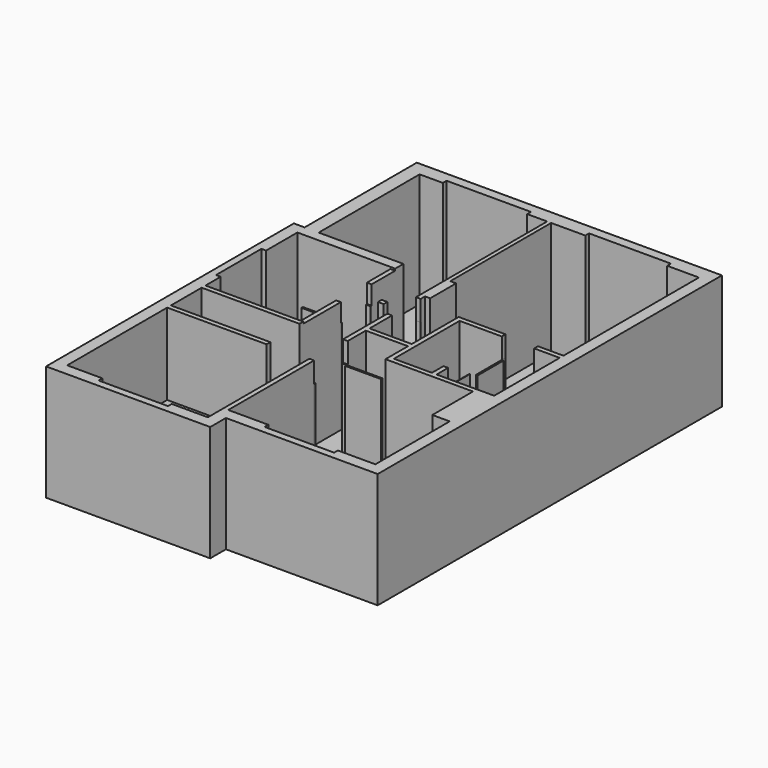
from build123d import *

# Parameters (mm, degrees)
F6_DEPTH  = 2440
F7_DEPTH  = 25
F8_DEPTH  = 2440
F2_W      = 100
F2_H      = 762
F9_DEPTH  = 3100
F3_W      = 690
F3_H      = 100
F10_DEPTH = 3100
F5_W      = 100
F5_H      = 1000
F5_H_2    = 627
F11_DEPTH = 2400
F12_W     = 10
F12_H     = 1000
F13_DEPTH = 2000
F14_W     = 600
F14_H     = 305
F15_DEPTH = 800
F18_DEPTH = 400
F19_W     = 600
F19_H     = 305
F20_DEPTH = 800
F22_DEPTH = 170
F23_W     = 30
F23_H     = 100
F24_DEPTH = 2000
F23_W_2   = 38
F23_H_2   = 762
F23_W_3   = 122
F25_W     = 100
F25_H     = 30
F26_DEPTH = 2000
F25_W_2   = 762
F25_H_2   = 38
F27_W     = 100
F27_H     = 30
F28_DEPTH = 2000
F27_W_2   = 762
F27_H_2   = 38
F29_W     = 760
F29_H     = 38
F30_DEPTH = 2000
F29_W_2   = 100
F29_H_2   = 30
F29_H_3   = 43.9612102509
F31_W     = 38
F31_H     = 690
F32_DEPTH = 2000
F31_W_2   = 30
F31_H_2   = 100
F33_W     = 1746.4833408594
F33_H     = 832.062959671
F34_DEPTH = 500
F35_W     = 906
F35_H     = 774.5329933167
F36_DEPTH = 706
F37_W     = 800
F37_H     = 1700
F38_DEPTH = 25
F40_DEPTH = 400


with BuildPart() as f6:
    # F0 (on Top) → F6 (new body)
    with BuildSketch(Plane.XY):
        Polygon((3250, -250), (3250, 168), (3704, 168), (5687, 168), (6486, 168), (6486, 2650), (6486, 3335), (6486, 9343), (775, 9343), (-20, 9343), (-20, 6353), (-250, 6353), (-250, -250), (499, -250), (2479, -250), align=None)
        Polygon((749, 0), (0, 0), (0, 2665), (6.1189043336, 2665), (2119, 2665), (2119, 2765), (0, 2765), (0, 3585), (2086, 3585), (2086, 3685), (1, 3685), (1, 4091), (-99, 4091), (-99, 5299), (1, 5299), (1, 6134), (2086, 6134), (2086, 6353), (280, 6353), (280, 9043), (775, 9043), (775, 9143), (2575, 9143), (2575, 9043), (3000, 9043), (3000, 3603), (3100, 3603), (3100, 5663), (3210, 5663), (3210, 6354), (3085, 6354), (3085, 9043), (3814, 9043), (3814, 9143), (5559, 9143), (5559, 9043), (6236, 9043), (6236, 3585), (5866, 3585), (5866, 2400), (6236, 2400), (6236, 418), (5437, 418), (5437, 318), (3954, 318), (3954, 418), (3100, 418), (3100, 2705), (3000, 2705), (3000, 0), (2229, 0), (2229, -100), (749, -100), align=None, mode=Mode.SUBTRACT)
    extrude(amount=F6_DEPTH)

    # F1 (on face) + F0 (on Top) → F7 (join)
    with BuildSketch(Plane.XY):
        Polygon((3100, 4183), (3100, 4083), (4000, 4083), (4000, 3483), (5866, 3483), (5866, 3583), (5010, 3583), (5010, 3890), (4910, 3890), (4910, 3583), (4100, 3583), (4100, 5333), (6236, 5333), (6236, 5433), (4000, 5433), (4000, 4183), align=None)
    with BuildSketch(Plane.XY):
        Polygon((3250, -250), (3250, 168), (3704, 168), (5687, 168), (6486, 168), (6486, 2650), (6486, 3335), (6486, 9343), (775, 9343), (-20, 9343), (-20, 6353), (-250, 6353), (-250, -250), (499, -250), (2479, -250), align=None)
        Polygon((749, 0), (0, 0), (0, 2665), (6.1189043336, 2665), (2119, 2665), (2119, 2765), (0, 2765), (0, 3585), (2086, 3585), (2086, 3685), (1, 3685), (1, 4091), (-99, 4091), (-99, 5299), (1, 5299), (1, 6134), (2086, 6134), (2086, 6353), (280, 6353), (280, 9043), (775, 9043), (775, 9143), (2575, 9143), (2575, 9043), (3000, 9043), (3000, 3603), (3100, 3603), (3100, 5663), (3210, 5663), (3210, 6354), (3085, 6354), (3085, 9043), (3814, 9043), (3814, 9143), (5559, 9143), (5559, 9043), (6236, 9043), (6236, 3585), (5866, 3585), (5866, 2400), (6236, 2400), (6236, 418), (5437, 418), (5437, 318), (3954, 318), (3954, 418), (3100, 418), (3100, 2705), (3000, 2705), (3000, 0), (2229, 0), (2229, -100), (749, -100), align=None, mode=Mode.SUBTRACT)
        Polygon((0, 2665), (0, 0), (749, 0), (749, -100), (2229, -100), (2229, 0), (3000, 0), (3000, 2705), (3100, 2705), (3100, 418), (3954, 418), (3954, 318), (5437, 318), (5437, 418), (6236, 418), (6236, 2400), (5866, 2400), (5866, 3585), (6236, 3585), (6236, 9043), (5559, 9043), (5559, 9143), (3814, 9143), (3814, 9043), (3085, 9043), (3085, 6354), (3210, 6354), (3210, 5663), (3100, 5663), (3100, 3603), (3000, 3603), (3000, 9043), (2575, 9043), (2575, 9143), (775, 9143), (775, 9043), (280, 9043), (280, 6353), (2086, 6353), (2086, 6134), (1, 6134), (1, 5299), (-99, 5299), (-99, 4091), (1, 4091), (1, 3685), (2086, 3685), (2086, 3585), (0, 3585), (0, 2765), (2119, 2765), (2119, 2665), (6.1189043336, 2665), align=None)
    extrude(amount=-F7_DEPTH)

    # F1 (on face) → F8 (join)
    with BuildSketch(Plane.XY):
        Polygon((3100, 4183), (3100, 4083), (4000, 4083), (4000, 3483), (5866, 3483), (5866, 3583), (5010, 3583), (5010, 3890), (4910, 3890), (4910, 3583), (4100, 3583), (4100, 5333), (6236, 5333), (6236, 5433), (4000, 5433), (4000, 4183), align=None)
    extrude(amount=F8_DEPTH)

    # F2 (on Top) → F9 (cut)
    with BuildSketch(Plane.XY):
        with Locations((3050, 5164)):
            Rectangle(F2_W, F2_H)
    extrude(amount=F9_DEPTH, mode=Mode.SUBTRACT)

    # F3 (on Top) → F10 (cut)
    with BuildSketch(Plane.XY):
        with Locations((5345, 5383)):
            Rectangle(F3_W, F3_H)
    extrude(amount=F10_DEPTH, mode=Mode.SUBTRACT)

    # F5 (on Top) → F11 (join)
    with BuildSketch(Plane.XY):
        with Locations((2036, 4185)):
            Rectangle(F5_W, F5_H)
        with Locations((2036, 5820.5)):
            Rectangle(F5_W, F5_H_2)
    extrude(amount=F11_DEPTH)

    # F12 (on Top) → F13 (join)
    with BuildSketch(Plane.XY):
        with Locations((4900, 4108)):
            Rectangle(F12_W, F12_H)
    extrude(amount=F13_DEPTH)

    # F14 (on Top) → F15 (join)
    with BuildSketch(Plane.XY):
        with Locations((5936, 3737.5)):
            Rectangle(F14_W, F14_H)
    extrude(amount=F15_DEPTH)

    # F17 (on Top) → F18 (join)
    with BuildSketch(Plane.XY):
        with BuildLine():
            ThreePointArc((5798.5, 4446), (5713.6471862576, 4410.8528137424), (5678.5, 4326))
            Line((5678.5, 4326), (5678.5, 3891))
            Line((5678.5, 3891), (6043.5, 3891))
            Line((6043.5, 3891), (6043.5, 4326))
            ThreePointArc((6043.5, 4326), (6008.3528137424, 4410.8528137424), (5923.5, 4446))
            Line((5923.5, 4446), (5798.5, 4446))
        make_face()
    extrude(amount=F18_DEPTH)

    # F35 (on Top) → F36 (join)
    with BuildSketch(Plane.XY):
        with Locations((453, 2279.2664966583)):
            Rectangle(F35_W, F35_H)
    extrude(amount=F36_DEPTH)

    # F37 (on Top) → F38 (join)
    with BuildSketch(Plane.XY):
        with Locations((4505, 4458)):
            Rectangle(F37_W, F37_H)
    extrude(amount=F38_DEPTH)

    # F39 (on Top) → F40 (join)
    with BuildSketch(Plane.XY):
        with BuildLine():
            Line((588.2481354475, 5527.7135048552), (588.2481354475, 5787.7135048552))
            ThreePointArc((588.2481354475, 5787.7135048552), (553.1009491899, 5872.5663185976), (468.2481354475, 5907.7135048552))
            Line((468.2481354475, 5907.7135048552), (133.2481354475, 5907.7135048552))
            Line((133.2481354475, 5907.7135048552), (133.2481354475, 5407.7135048552))
            Line((133.2481354475, 5407.7135048552), (468.2481354475, 5407.7135048552))
            ThreePointArc((468.2481354475, 5407.7135048553), (553.1009491899, 5442.8606911129), (588.2481354475, 5527.7135048552))
        make_face()
        with BuildLine():
            Line((708.5185599327, 5154.1996002197), (133.2481354475, 5154.1996002197))
            Line((133.2481354475, 5154.1996002197), (133.2481354475, 4828.3729553223))
            Line((133.2481354475, 4828.3729553223), (708.5185599327, 4828.3729553223))
            ThreePointArc((708.5185599327, 4828.3729553223), (722.6606955564, 4834.2308196985), (728.5185599327, 4848.3729553223))
            Line((728.5185599327, 4848.3729553223), (728.5185599327, 5134.1996002197))
            ThreePointArc((728.5185599327, 5134.1996002197), (722.6606955564, 5148.3417358435), (708.5185599327, 5154.1996002197))
        make_face()
    extrude(amount=F40_DEPTH)


with BuildPart() as f20:
    # F19 (on Top) → F20 (new body)
    with BuildSketch(Plane.XY):
        with Locations((5336, 3737.5)):
            Rectangle(F19_W, F19_H)
    extrude(amount=F20_DEPTH)

    # F21 (on face) → F22 (join)
    with BuildSketch(Plane.XY.offset(800)):
        with BuildLine():
            Line((5466, 4065), (5206, 4065))
            ThreePointArc((5206, 4065), (5121.1471862576, 4029.8528137424), (5086, 3945))
            Line((5086, 3945), (5086, 3610))
            Line((5086, 3610), (5586, 3610))
            Line((5586, 3610), (5586, 3945))
            ThreePointArc((5586, 3945), (5550.8528137424, 4029.8528137424), (5466, 4065))
        make_face()
    extrude(amount=-F22_DEPTH)


with BuildPart() as f24:
    # F23 (on Top) → F24 (new body)
    with BuildSketch(Plane.XY):
        with Locations((2985, 5713)):
            Rectangle(F23_W, F23_H)
    extrude(amount=F24_DEPTH)


with BuildPart() as f24b:
    # F23 (on Top) → F24, piece 2 (new body)
    with BuildSketch(Plane.XY):
        with Locations((2951, 6144)):
            Rectangle(F23_W_2, F23_H_2)
    extrude(amount=F24_DEPTH)


with BuildPart() as f24c:
    # F23 (on Top) → F24, piece 3 (new body)
    with BuildSketch(Plane.XY):
        with Locations((2147, 5725.5080223083)):
            Rectangle(F23_W_3, F23_H)
    extrude(amount=F24_DEPTH)


with BuildPart() as f26:
    # F25 (on Top) → F26 (new body)
    with BuildSketch(Plane.XY):
        with Locations((2036, 4700)):
            Rectangle(F25_W, F25_H)
    extrude(amount=F26_DEPTH)


with BuildPart() as f26b:
    # F25 (on Top) → F26, piece 2 (new body)
    with BuildSketch(Plane.XY):
        with Locations((1605, 4734)):
            Rectangle(F25_W_2, F25_H_2)
    extrude(amount=F26_DEPTH)


with BuildPart() as f26c:
    # F25 (on Top) → F26, piece 3 (new body)
    with BuildSketch(Plane.XY):
        with Locations((2036, 5492)):
            Rectangle(F25_W, F25_H)
    extrude(amount=F26_DEPTH)


with BuildPart() as f28:
    # F27 (on Top) → F28 (new body)
    with BuildSketch(Plane.XY):
        with Locations((3050, 5560)):
            Rectangle(F27_W, F27_H)
    extrude(amount=F28_DEPTH)


with BuildPart() as f28b:
    # F27 (on Top) → F28, piece 2 (new body)
    with BuildSketch(Plane.XY):
        Polygon((3100, 4783), (3000, 4783), (3000, 4685.0380897522), (3100, 4685.0380897522), (3100, 4723.0380897522), align=None)
        with Locations((3481, 4704.0380897522)):
            Rectangle(F27_W_2, F27_H_2)
    extrude(amount=F28_DEPTH)


with BuildPart() as f30:
    # F29 (on Top) → F30 (new body)
    with BuildSketch(Plane.XY):
        with Locations((3480, 3554)):
            Rectangle(F29_W, F29_H)
    extrude(amount=F30_DEPTH)


with BuildPart() as f30b:
    # F29 (on Top) → F30, piece 2 (new body)
    with BuildSketch(Plane.XY):
        with Locations((3050, 3588)):
            Rectangle(F29_W_2, F29_H_2)
    extrude(amount=F30_DEPTH)


with BuildPart() as f30c:
    # F29 (on Top) → F30, piece 3 (new body)
    with BuildSketch(Plane.XY):
        with Locations((3050, 2726.9806051254)):
            Rectangle(F29_W_2, F29_H_3)
    extrude(amount=F30_DEPTH)


with BuildPart() as f32:
    # F31 (on face) → F32 (new body)
    with BuildSketch(Plane.XY):
        with Locations((5019, 4988)):
            Rectangle(F31_W, F31_H)
    extrude(amount=F32_DEPTH)


with BuildPart() as f32b:
    # F31 (on face) → F32, piece 2 (new body)
    with BuildSketch(Plane.XY):
        with Locations((4985, 5383)):
            Rectangle(F31_W_2, F31_H_2)
    extrude(amount=F32_DEPTH)


with BuildPart() as f32c:
    # F31 (on face) → F32, piece 3 (new body)
    with BuildSketch(Plane.XY):
        with Locations((5705, 5383)):
            Rectangle(F31_W_2, F31_H_2)
    extrude(amount=F32_DEPTH)


with BuildPart() as f34:
    # F33 (on Top) → F34 (new body)
    with BuildSketch(Plane.XY):
        with Locations((1062.913171947, 4161.8102788925)):
            Rectangle(F33_W, F33_H)
        with BuildLine():
            ThreePointArc((392.0536339283, 4437.9125785828), (414.0206253393, 4490.9455871718), (467.0536339283, 4512.9125785828))
            Line((467.0536339283, 4512.9125785828), (1838.7377691269, 4512.9125785828))
            Line((1838.7377691269, 4512.9125785828), (1838.7377691269, 3820.7157421112))
            Line((1838.7377691269, 3820.7157421112), (467.0536339283, 3820.7157421112))
            ThreePointArc((467.0536339283, 3820.7157421112), (414.0206253393, 3842.6827335222), (392.0536339283, 3895.7157421112))
            Line((392.0536339283, 3895.7157421112), (392.0536339283, 4437.9125785828))
        make_face(mode=Mode.SUBTRACT)
    extrude(amount=F34_DEPTH)


solid = Compound([f6.part, f20.part, f24.part, f24b.part, f24c.part, f26.part, f26b.part, f26c.part, f28.part, f28b.part, f30.part, f30b.part, f30c.part, f32.part, f32b.part, f32c.part, f34.part])
